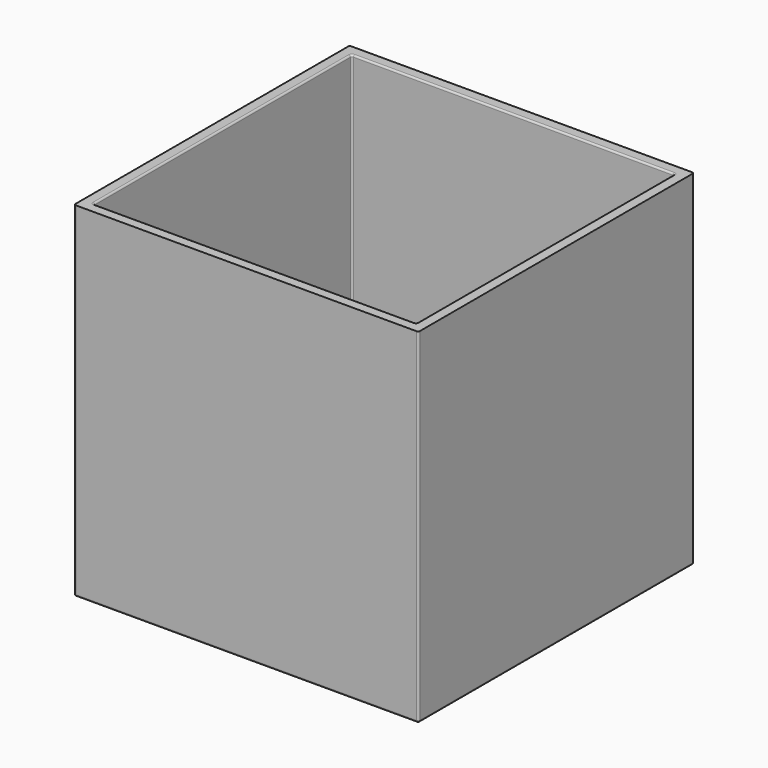
from build123d import *

# Parameters (mm, degrees)
F0_W         = 50.8
F0_H         = 50.8
F1_DEPTH     = 1.5875
F2_W         = 50.8
F2_H         = 50.8
F2_W_2       = 47.625
F2_H_2       = 47.625
F3_DEPTH     = 49.2125
F4_R         = 0.254
F5_TEXT_SIZE = 3.7101570244
F6_DEPTH     = 0.254


# Not quite as in the source:
# - Text() gives the source's letters only with a copy of the font that has no kerning and outlines rounded to 1/6400 em; it was checked with that copy


with BuildPart() as f1:
    # F0 (on Top) → F1 (new body)
    with BuildSketch(Plane.XY):
        Rectangle(F0_W, F0_H)
    extrude(amount=F1_DEPTH)

    # F2 (on face) → F3 (join)
    with BuildSketch(Plane.XY.offset(1.5875)):
        Rectangle(F2_W, F2_H)
        Rectangle(F2_W_2, F2_H_2, mode=Mode.SUBTRACT)
    extrude(amount=F3_DEPTH)

    # F4
    f4_edges = [f1.edges().sort_by_distance(p)[0] for p in [
        (-23.8125, 0, 1.5875),
        (-23.8125, -23.8125, 26.19375),
        (0, -23.8125, 1.5875),
        (-23.8125, 0, 50.8),
        (0, -23.8125, 50.8),
        (0, 23.8125, 1.5875),
        (-23.8125, 23.8125, 26.19375),
        (0, 23.8125, 50.8),
        (23.8125, 23.8125, 26.19375),
        (23.8125, 0, 1.5875),
        (23.8125, 0, 50.8),
        (23.8125, -23.8125, 26.19375),
        (-25.4, -25.4, 25.4),
        (25.4, -25.4, 25.4),
        (25.4, 25.4, 25.4),
        (-25.4, 25.4, 25.4),
        (-25.4, 0, 0),
        (0, -25.4, 0),
        (0, 25.4, 0),
        (25.4, 0, 0),
    ]]
    fillet(f4_edges, radius=F4_R)

    # F5 (on face) → F6 (cut)
    with BuildSketch(Plane(origin=(0, 25.4, 0), x_dir=(-1, 0, 0), z_dir=(0, 1, 0))):
        with Locations((-22.225, 35.4286869425)):
            Text('2-Prong PWM Connectors', F5_TEXT_SIZE, font='Open Sans', text_align=(TextAlign.LEFT, TextAlign.BOTTOM))
    extrude(amount=-F6_DEPTH, mode=Mode.SUBTRACT)


solid = f1.part
